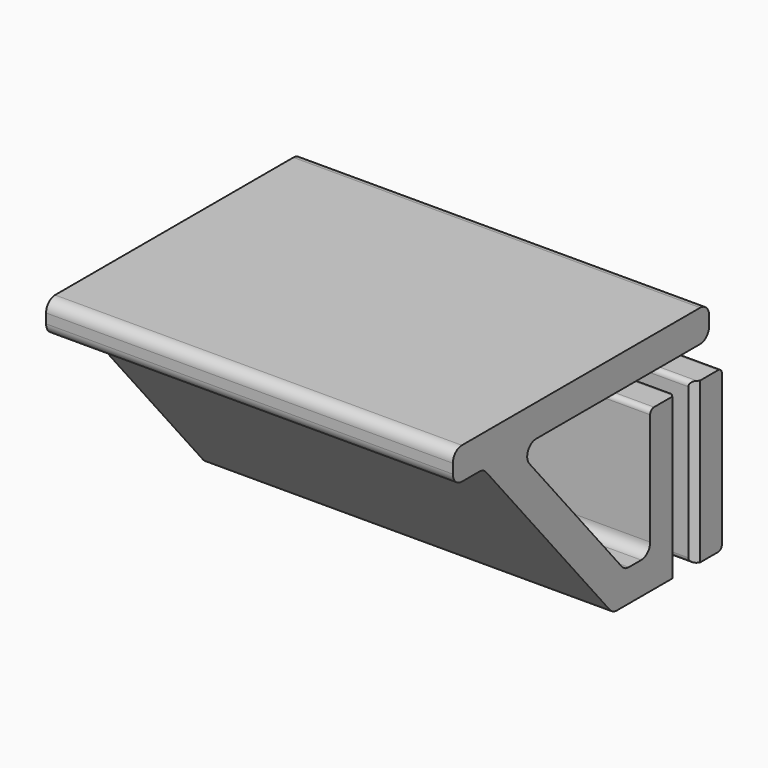
from build123d import *

# Parameters (mm, degrees)
F0_W     = 25.4
F0_H     = 5.6
F1_DEPTH = 10
F2_W     = 4.6
F2_H     = 1.35
F3_DEPTH = 10
F5_DEPTH = 5.6
F7_DEPTH = 25.4
F8_SIZE  = 0.4
F9_R     = 0.7
F10_R    = 0.29999


# Not quite as in the source:
# - a fillet or chamfer is up to 0.001 mm smaller than in the source, because OpenCascade refuses the exact size


with BuildPart() as f1:
    # F0 (on Top) → F1 (new body)
    with BuildSketch(Plane.XY):
        Rectangle(F0_W, F0_H)
    extrude(amount=F1_DEPTH)

    # F2 (on face) → F3 (cut, through all)
    with BuildSketch(Plane.XY.offset(10)):
        with Locations((-10.4, 0)):
            Rectangle(F2_W, F2_H)
        with Locations((10.4, 0)):
            Rectangle(F2_W, F2_H)
    extrude(amount=-F3_DEPTH, mode=Mode.SUBTRACT)

    # F4 (on face) → F5 (cut, through all)
    with BuildSketch(Plane.XZ.offset(2.8)):
        Polygon((6, 10), (-6, 10), (-1, 3), (1, 3), align=None)
    extrude(amount=-F5_DEPTH, mode=Mode.SUBTRACT)

    # F6 (on face) → F7 (join, through all)
    with BuildSketch(Plane(origin=(-12.7, 0, 0), x_dir=(0, -1, 0), z_dir=(-1, 0, 0))):
        Polygon((2.8, 2), (2.8, 0), (5.7319724348, 0), (15.8119724348, 12), (18.2, 12), (18.2, 14), (-1.8, 14), (-1.8, 12), (13.2, 12), (4.8, 2), align=None)
    extrude(amount=-F7_DEPTH)

    # F8
    f8_edges = [f1.edges().sort_by_distance(p)[0] for p in [
        (12.7, 0.675, 5),
        (12.7, -0.675, 5),
    ]]
    chamfer(f8_edges, length=F8_SIZE)

    # F9
    f9_edges = [f1.edges().sort_by_distance(p)[0] for p in [
        (0, -2.8, 2),
        (0, -4.8, 2),
        (0, -13.2, 12),
        (0, -15.811972, 12),
        (0, -5.731972, 0),
        (0, -18.2, 12),
        (0, -18.2, 14),
        (0, 1.8, 12),
        (0, 1.8, 14),
    ]]
    fillet(f9_edges, radius=F9_R)

    # F10 (radius 0.3 in the source; OpenCascade refuses exactly that, so slightly less here)
    f10_edges = [f1.edges().sort_by_distance(p)[0] for p in [
        (0, 2.8, 0),
        (9.35, 2.8, 10),
        (-9.35, 2.8, 10),
        (-10.4, 0.675, 0),
        (10.2, 0.675, 0),
        (10.2, -0.675, 0),
        (-10.4, -0.675, 0),
        (10.2, 0.675, 10),
        (10.2, -0.675, 10),
        (9.35, -2.8, 10),
        (-10.4, 0.675, 10),
        (-10.4, -0.675, 10),
        (-9.35, -2.8, 10),
        (3.5, 2.8, 6.5),
        (0, 2.8, 3),
        (-3.5, 2.8, 6.5),
        (0, -2.8, 3),
        (3.5, -2.8, 6.5),
        (-3.5, -2.8, 6.5),
    ]]
    fillet(f10_edges, radius=F10_R)


solid = f1.part
